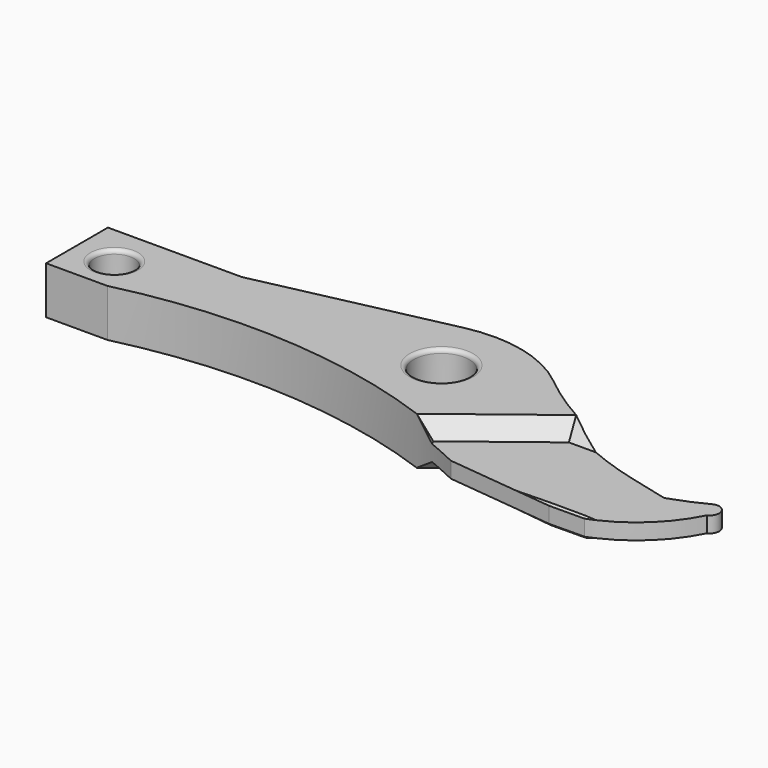
from build123d import *

# Parameters (mm, degrees)
F0_R     = 2.5
F0_R_2   = 3.5
F1_DEPTH = 3
F2_SIZE  = 2
F4_R     = 0.5
F5_DEPTH = 2
F5_TAPER = 45


# Not quite as in the source:
# - a pattern or mirror of a feature is missing from the dataset's text; its kind, count and spacing are read off the source's solid


with BuildPart() as f1:
    # F0 (on Top) → F1 (new body, symmetric)
    with BuildSketch(Plane.XY):
        with BuildLine():
            Line((-22.6589401231, 2.4236629568), (-39.5600539291, 2.4236629568))
            Line((-39.5600539291, 2.4236629568), (-39.5600539291, -7.3263370432))
            Line((-39.5600539291, -7.3263370432), (-31.8100539291, -7.3263370432))
            ThreePointArc((-31.8100539291, -7.3263370432), (-7.74599031, -5.7290436956), (15.4584982429, -12.300361288))
            Line((15.4584982429, -12.300361288), (29.0535219773, -13.773592777))
            Line((29.0535219773, -13.773592777), (33.4806282794, -13.7333460718))
            ThreePointArc((33.4806282794, -13.7333460718), (38.7220078669, -10.5438462203), (42.4399460709, -5.663077347))
            ThreePointArc((42.4399460709, -5.663077347), (43.0076744864, -4.0355880404), (41.3801851798, -3.4678596249))
            Line((41.3801851798, -3.4678596249), (39.4420786101, -4.4034978191))
            Line((39.4420786101, -4.4034978191), (36.8522457248, -5.3948726996))
            Line((36.8522457248, -5.3948726996), (31.776658302, -4.1156165412))
            ThreePointArc((31.776658302, -4.1156165412), (22.9700739727, -0.8151163334), (15.0904607998, 4.3191728497))
            ThreePointArc((15.0904607998, 4.3191728497), (8.5263135264, 7.5598223627), (1.2061465951, 7.6304961974))
            Line((1.2061465951, 7.6304961974), (-22.6589401231, 2.4236629568))
        make_face()
        with Locations((-34.5600539291, -2.8220066844)):
            Circle(F0_R, mode=Mode.SUBTRACT)
        with Locations((4.4399460709, 0)):
            Circle(F0_R_2, mode=Mode.SUBTRACT)
    extrude(amount=F1_DEPTH, both=True)

    # F2
    f2_edges = [f1.edges().sort_by_distance(p)[0] for p in [
        (22.25601, -13.036977, 3),
        (22.25601, -13.036977, -3),
        (31.267075, -13.753469, 3),
        (31.267075, -13.753469, -3),
        (38.722008, -10.543846, 3),
        (38.722008, -10.543846, -3),
    ]]
    chamfer(f2_edges, length=F2_SIZE)

    # F4
    f4_edges = [f1.edges().sort_by_distance(p)[0] for p in [
        (0.939946, 0, -3),
        (-37.060054, -2.822007, -3),
        (-37.060054, -2.822007, 3),
        (0.939946, 0, 3),
    ]]
    fillet(f4_edges, radius=F4_R)

    # F3 (on face) → F5 (cut)
    with BuildSketch(Plane(origin=(0, 0, -3), x_dir=(1, 0, 0), z_dir=(0, 0, -1))):
        Polygon((11.9156481301, 15.2815678021), (9.0032261915, 9.5891237242), (21.4353172765, 0), (52.8852939606, 0), (52.8852939606, 15.2815678021), align=None)
    f5 = extrude(amount=-F5_DEPTH, taper=F5_TAPER, mode=Mode.SUBTRACT)

    # F5_copies: F5 across plane
    add(f5.mirror(Plane.XY), mode=Mode.SUBTRACT)


solid = f1.part
